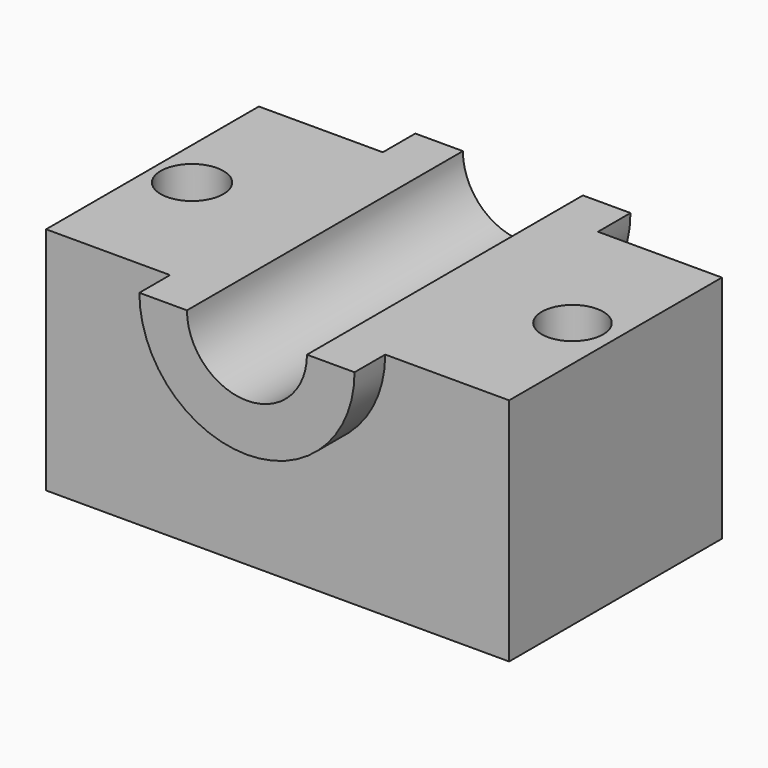
from build123d import *

# Parameters (mm, degrees)
F0_W     = 153.4594595432
F0_H     = 88.1393551826
F2_DEPTH = 76.2
F1_R     = 10.1701349395
F1_R_2   = 10.3995540655
F3_DEPTH = 76.201
F5_DEPTH = 101.6
F7_DEPTH = 12.7
F9_DEPTH = 114.301


with BuildPart() as f2:
    # F0 (on Top) → F2 (new body)
    with BuildSketch(Plane.XY):
        Rectangle(F0_W, F0_H)
    extrude(amount=F2_DEPTH)

    # F1 (on face) → F3 (cut, through all)
    with BuildSketch(Plane.XY):
        with Locations((62.4677017331, 0)):
            Circle(F1_R)
        with Locations((-63.608661294, 0)):
            Circle(F1_R_2)
    extrude(amount=F3_DEPTH, mode=Mode.SUBTRACT)

    # F4 (on face) → F5 (join)
    with BuildSketch(Plane.XZ.offset(44.0696775913)):
        with BuildLine():
            ThreePointArc((-35.6539782969, 76.2), (0, 40.5460217031), (35.6539782969, 76.2))
            Line((35.6539782969, 76.2), (-35.6539782969, 76.2))
        make_face()
    extrude(amount=-F5_DEPTH)

    # F6 (on face) → F7 (join)
    with BuildSketch(Plane.XZ.offset(44.0696775913)):
        with BuildLine():
            ThreePointArc((-35.6539782969, 76.2), (0, 40.5460217031), (35.6539782969, 76.2))
            Line((35.6539782969, 76.2), (-35.6539782969, 76.2))
        make_face()
    extrude(amount=F7_DEPTH)

    # F8 (on face) → F9 (cut, through all)
    with BuildSketch(Plane.XZ.offset(56.7696775913)):
        with BuildLine():
            ThreePointArc((-19.8833374867, 76.2), (0, 56.3166625133), (19.8833374867, 76.2))
            Line((19.8833374867, 76.2), (-19.8833374867, 76.2))
        make_face()
        with BuildLine():
            Line((-19.8833374867, 76.2), (19.8833374867, 76.2))
            ThreePointArc((19.8833374867, 76.2), (0, 96.0833374867), (-19.8833374867, 76.2))
        make_face()
    extrude(amount=-F9_DEPTH, mode=Mode.SUBTRACT)


solid = f2.part
